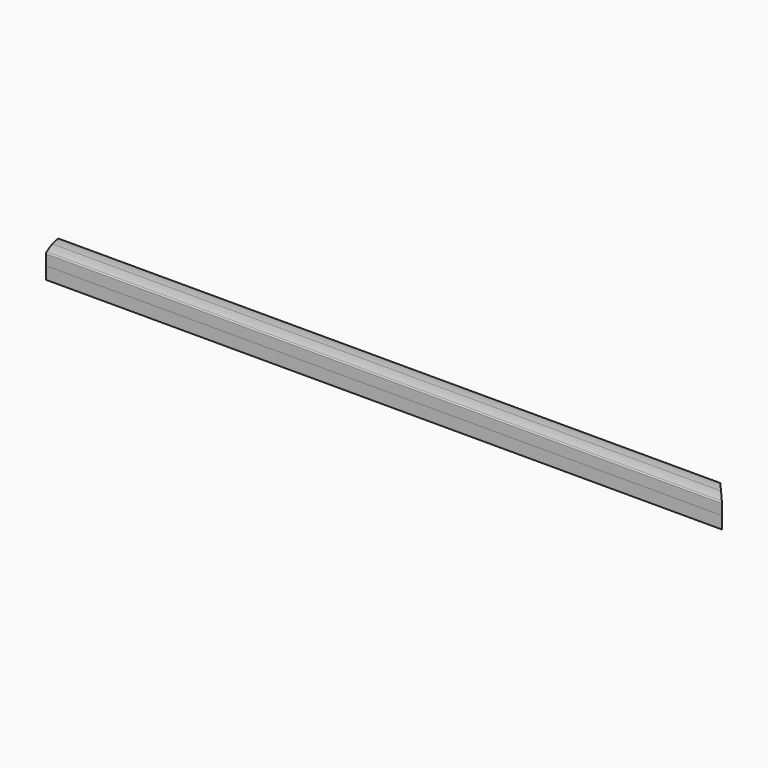
from build123d import *

# Parameters (mm, degrees)
F2_DEPTH      = 1000
F4_DEPTH      = 1000
F8_DEPTH      = 10.001
F8_DEPTH_BACK = 10.001


with BuildPart() as f2:
    # F1 (on Right) → F2 (new body)
    with BuildSketch(Plane.YZ):
        with BuildLine():
            Line((0, -9), (0, -10))
            Line((0, -10), (10, -10))
            Line((10, -10), (10, -0.2))
            Line((10, -0.2), (9, -0.2))
            ThreePointArc((9, -0.2), (8.5, -0.7), (9, -1.2))
            ThreePointArc((9, -1.2), (9.5, -1.7), (9, -2.2))
            Line((9, -2.2), (9, -9))
            Line((9, -9), (0, -9))
        make_face()
    extrude(amount=F2_DEPTH)

    # F5: F2 across plane


with BuildPart() as f4:
    # F3 (on Right) → F4 (new body)
    with BuildSketch(Plane.YZ):
        with BuildLine():
            Line((9, -0.2), (10, -0.2))
            Line((10, -0.2), (10, 8.1663783152))
            ThreePointArc((10, 8.1663783152), (9.7693092582, 8.8052548802), (9.1836734694, 9.1493656277))
            ThreePointArc((9.1836734694, 9.1493656277), (4.6114920912, 9.7868872364), (0, 10))
            Line((0, 10), (0, 9))
            ThreePointArc((0, 9), (4.5192622493, 8.7911494917), (9, 8.1663783152))
            Line((9, 8.1663783152), (9, 0.8))
            ThreePointArc((9, 0.8), (7.5, -0.7), (9, -2.2))
            ThreePointArc((9, -2.2), (9.5, -1.7), (9, -1.2))
            ThreePointArc((9, -1.2), (8.5, -0.7), (9, -0.2))
        make_face()
    extrude(amount=F4_DEPTH)

    # F6: F4 across plane


with BuildPart() as f2_1:
    add(f2.part)
    add(f2.part.mirror(Plane.XZ))


with BuildPart() as f4_1:
    add(f4.part)
    add(f4.part.mirror(Plane.XZ))


with BuildPart() as f8_tool:
    # F7 (on Top) → F8 (new body, two sides)
    with BuildSketch(Plane.XY) as f8_sk:
        Polygon((0, 10), (0, 0), (0, -10), (6.0383560074, -10), align=None)
        Polygon((709.9114181152, 10), (524.652621251, 10), (542.0383560074, -10), (1016.9613361359, -10), (1016.9613361359, 10), align=None)
    extrude(amount=F8_DEPTH)
    extrude(f8_sk.sketch, amount=-F8_DEPTH_BACK)


with BuildPart() as f2_2:
    add(f2_1.part)

    # F8: cut by f8_tool
    add(f8_tool.part, mode=Mode.SUBTRACT)


with BuildPart() as f4_2:
    add(f4_1.part)

    # F8: cut by f8_tool
    add(f8_tool.part, mode=Mode.SUBTRACT)


solid = Compound([f2_2.part, f4_2.part])
